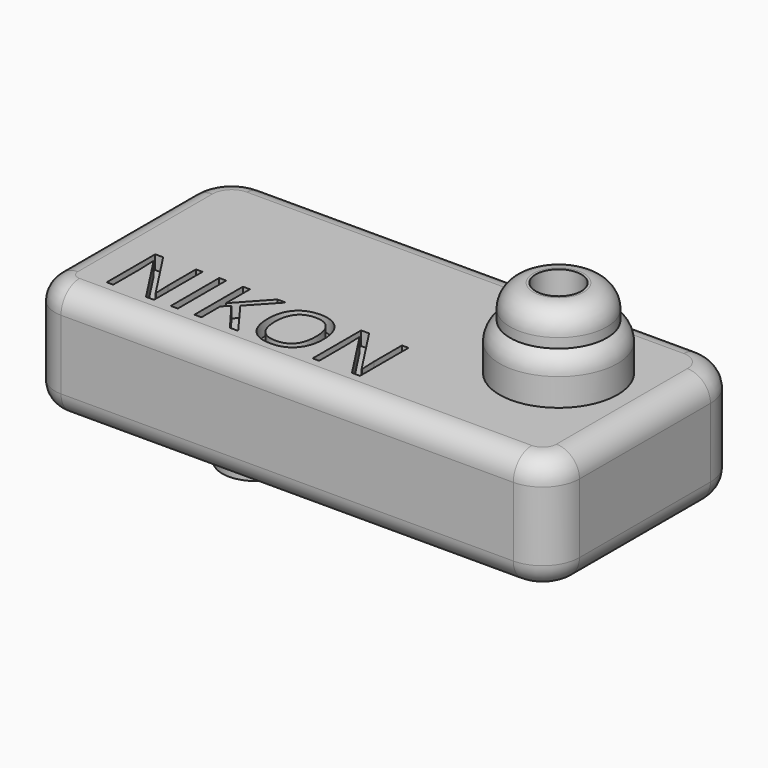
from build123d import *

# Parameters (mm, degrees)
F0_W          = 112.735144794
F0_H          = 52.3730162531
F1_DEPTH      = 25
F2_R          = 12.792638752
F3_DEPTH      = 10.1
F4_R          = 10.4881187531
F5_DEPTH      = 7.1
F6_R          = 6.2364428887
F7_DEPTH      = 6.3
F8_R          = 5.527092149
F9_DEPTH      = 6.8
F10_R         = 4.9401962669
F11_DEPTH     = 25
F12_R         = 9.174011537
F13_R         = 8.9325901808
F14_R         = 7.9669047558
F15_R         = 6.7597979746
F16_R         = 4.1517104059
F17_DEPTH     = 2.7
F19_R         = 5
F20_W         = 36.9829768315
F20_H         = 18.6613015831
F21_DEPTH     = 4
F22_R         = 5
F23_R         = 5
F24_TEXT_SIZE = 18.4035713743
F25_DEPTH     = 3
F26_R         = 7.4599315502
F27_DEPTH     = 5.6
F28_R         = 7.2012794592
F29_DEPTH     = 4.9


# Not quite as in the source:
# - a fillet or chamfer that OpenCascade refuses, or shapes differently, is made with other operations: its cross-section is extruded or revolved along the edge and cut away or added
# - Text() gives the source's letters only with a copy of the font that has no kerning and outlines rounded to 1/6400 em; it was checked with that copy


with BuildPart() as f1:
    # F0 (on Top) → F1 (new body)
    with BuildSketch(Plane.XY):
        with Locations((-3.1297281384, 0.5861828104)):
            Rectangle(F0_W, F0_H)
    extrude(amount=F1_DEPTH)

    # F2 (on face) → F3 (join)
    with BuildSketch(Plane.XY.offset(25)):
        with Locations((32.2079472244, 2.9800147749)):
            Circle(F2_R)
    extrude(amount=F3_DEPTH)

    # F4 (on face) → F5 (join)
    with BuildSketch(Plane.XY.offset(35.1)):
        with Locations((32.2079472244, 2.9800147749)):
            Circle(F4_R)
    extrude(amount=F5_DEPTH)

    # F6 (on face) → F7 (join)
    with BuildSketch(Plane.XY.offset(42.2)):
        with Locations((32.2079472244, 2.9800147749)):
            Circle(F6_R)
    extrude(amount=-F7_DEPTH)

    # F8 (on face) → F9 (join)
    with BuildSketch(Plane.XY.offset(42.2)):
        with Locations((32.2079472244, 2.9800147749)):
            Circle(F8_R)
    extrude(amount=-F9_DEPTH)

    # F10 (on face) → F11 (cut)
    with BuildSketch(Plane.XY.offset(42.2)):
        with Locations((32.2079472244, 2.9800147749)):
            Circle(F10_R)
    extrude(amount=-F11_DEPTH, mode=Mode.SUBTRACT)

    # F12
    f12_edges = [f1.edges().sort_by_distance(p)[0] for p in [
        (-59.497301, 26.772691, 12.5),
    ]]
    fillet(f12_edges, radius=F12_R)

    # F13
    f13_edges = [f1.edges().sort_by_distance(p)[0] for p in [
        (53.237844, 26.772691, 12.5),
    ]]
    fillet(f13_edges, radius=F13_R)

    # F14
    f14_edges = [f1.edges().sort_by_distance(p)[0] for p in [
        (53.237844, -25.600325, 12.5),
    ]]
    fillet(f14_edges, radius=F14_R)

    # F15
    f15_edges = [f1.edges().sort_by_distance(p)[0] for p in [
        (-59.497301, -25.600325, 12.5),
    ]]
    fillet(f15_edges, radius=F15_R)

    # F16 (on face) → F17 (join)
    with BuildSketch(Plane(origin=(0, 26.7726909369, 0), x_dir=(-1, 0, 0), z_dir=(0, 1, 0))):
        with Locations((43.6965599656, 10.9036965296)):
            Circle(F16_R)
    extrude(amount=F17_DEPTH)

    # F18: fillet of radius 5 on 1 edges, made by hand

    # F18_s1 → F18_t2 (revolve, cut)
    with BuildSketch(Plane.XZ.offset(-2.9800147749)):
        with BuildLine():
            ThreePointArc((45.0009859764, 30.8882499544), (44.3871394256, 33.2889445545), (42.6962816515, 35.1003368749))
            Line((42.6962816515, 35.1003368749), (42.9659477876, 35.521545567))
            ThreePointArc((42.9659477876, 35.521545567), (43.848433814, 35.6001365685), (45.0005859764, 35.6001365685))
            Line((45.0005859764, 35.6001365685), (45.5007225449, 35.1))
            ThreePointArc((45.5007225449, 35.1), (45.5007225449, 32.9941249772), (45.5011225449, 30.8882499544))
            Line((45.5011225449, 30.8882499544), (45.0009859764, 30.8882499544))
        make_face()
    revolve(axis=Axis((32.2079472244, 2.9800147749, 35.1), (0, 0, 1)), mode=Mode.SUBTRACT)

    # F19
    f19_edges = [f1.edges().sort_by_distance(p)[0] for p in [
        (21.719828, 2.980015, 42.2),
    ]]
    fillet(f19_edges, radius=F19_R)

    # F20 (on face) → F21 (join)
    with BuildSketch(Plane(origin=(0, 0, 0), x_dir=(1, 0, 0), z_dir=(0, 0, -1))):
        with Locations((13.9766852371, -0.490420498)):
            Rectangle(F20_W, F20_H)
    extrude(amount=F21_DEPTH)

    # F22
    f22_edges = [f1.edges().sort_by_distance(p)[0] for p in [
        (-3.009017, 26.772691, 25),
    ]]
    fillet(f22_edges, radius=F22_R)

    # F23
    f23_edges = [f1.edges().sort_by_distance(p)[0] for p in [
        (-3.009017, 26.772691, 0),
        (50.621549, 24.156396, 0),
        (-56.810295, 24.085685, 0),
        (53.237844, 0.10334, 0),
        (-59.497301, -0.620924, 0),
        (50.904392, -23.266873, 0),
        (-57.517402, -23.620426, 0),
        (-3.733282, -25.600325, 0),
    ]]
    fillet(f23_edges, radius=F23_R)

    # F24 (on face) → F25 (cut)
    with BuildSketch(Plane.XY.offset(25)):
        with Locations((-50.0526688993, -18.8405273415)):
            Text('NIKON', F24_TEXT_SIZE, font='Open Sans', text_align=(TextAlign.LEFT, TextAlign.BOTTOM))
    extrude(amount=-F25_DEPTH, mode=Mode.SUBTRACT)

    # F26 (on face) → F27 (join)
    with BuildSketch(Plane(origin=(0, 0, 0), x_dir=(1, 0, 0), z_dir=(0, 0, -1))):
        with Locations((-24.9888096005, -8.0204885453)):
            Circle(F26_R)
    extrude(amount=F27_DEPTH)

    # F28 (on face) → F29 (join)
    with BuildSketch(Plane(origin=(0, 0, 0), x_dir=(1, 0, 0), z_dir=(0, 0, -1))):
        with Locations((-23.4353709966, 9.5111588016)):
            Circle(F28_R)
    extrude(amount=F29_DEPTH)


solid = f1.part
